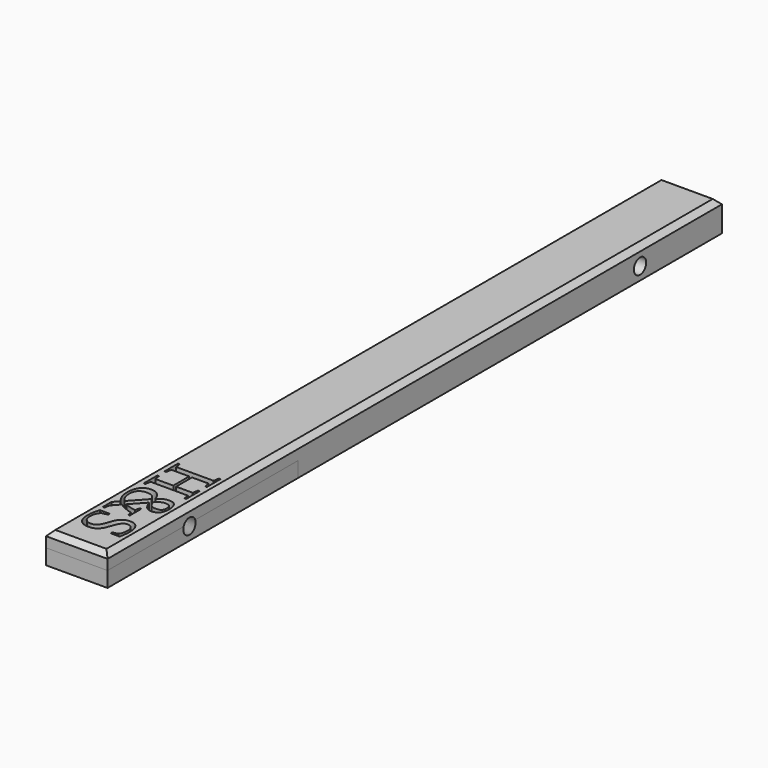
from build123d import *

# Parameters (mm, degrees)
F0_W         = 6
F0_H         = 75
F1_DEPTH     = 3
F2_TEXT_SIZE = 6.32074755
F3_DEPTH     = 28.9
F4_W         = 6
F4_H         = 23.268167302
F5_DEPTH     = 1.5
F6_SIZE      = 0.5
F7_SIZE      = 0.5
F8_SIZE      = 0.5
F9_R         = 0.75
F10_DEPTH    = 6.0010001


# Not quite as in the source:
# - Text() gives the source's letters only with a copy of the font that has no kerning and outlines rounded to 1/6400 em; it was checked with that copy


with BuildPart() as f1:
    # F0 (on Top) → F1 (new body)
    with BuildSketch(Plane.XY):
        with Locations((1.2593792815, -7.8569538891)):
            Rectangle(F0_W, F0_H)
    extrude(amount=F1_DEPTH)

    # F2 (on Top) → F3 (cut)
    with BuildSketch(Plane.XY):
        with Locations(Location((-0.7803445786, -30.2660847695), (0, 0, -90))):
            Text('H&S', F2_TEXT_SIZE, font='Tinos', text_align=(TextAlign.LEFT, TextAlign.BOTTOM))
    extrude(amount=F3_DEPTH, mode=Mode.SUBTRACT)

    # F6
    f6_edges = [f1.edges().sort_by_distance(p)[0] for p in [
        (-1.740621, -7.856954, 3),
        (4.259379, -7.856954, 3),
    ]]
    chamfer(f6_edges, length=F6_SIZE)

    # F7
    f7_edges = [f1.edges().sort_by_distance(p)[0] for p in [
        (1.259379, -45.356954, 3),
    ]]
    chamfer(f7_edges, length=F7_SIZE)

    # F8
    f8_edges = [f1.edges().sort_by_distance(p)[0] for p in [
        (1.259379, 29.643046, 3),
    ]]
    chamfer(f8_edges, length=F8_SIZE)


with BuildPart() as f5:
    # F4 (on face) → F5 (new body)
    with BuildSketch(Plane(origin=(0, 0, 0), x_dir=(1, 0, 0), z_dir=(0, 0, -1))):
        with Locations((1.2593792815, 33.7228702381)):
            Rectangle(F4_W, F4_H)
    extrude(amount=-F5_DEPTH)


with BuildPart() as f10_tool:
    # F9 (on face) → F10 (new body, through all)
    with BuildSketch(Plane.YZ.offset(4.2593792815)):
        with Locations((19.6430461109, 1.25)):
            Circle(F9_R)
        with Locations((-35.3569538891, 1.25)):
            Circle(F9_R)
    extrude(amount=-F10_DEPTH)


with BuildPart() as f1_1:
    add(f1.part)

    # F10: cut by f10_tool
    add(f10_tool.part, mode=Mode.SUBTRACT)


with BuildPart() as f5_1:
    add(f5.part)

    # F10: cut by f10_tool
    add(f10_tool.part, mode=Mode.SUBTRACT)


solid = Compound([f1_1.part, f5_1.part])
